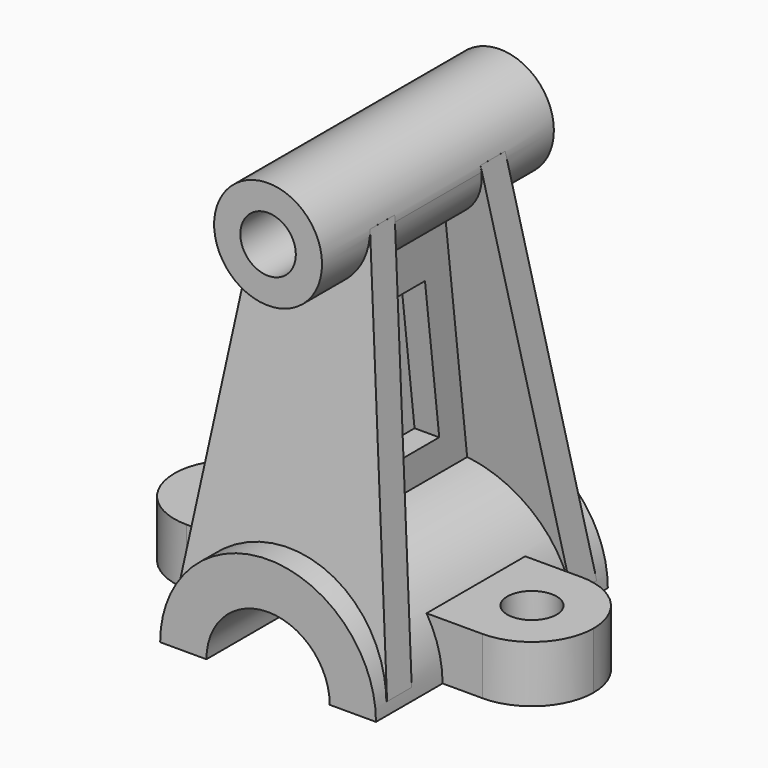
from build123d import *

# Parameters (mm, degrees)
F1_DEPTH     = 37.30625
F2_DEPTH     = 15.875
F3_R         = 15.87499
F0_R         = 13.890625
F0_R_2       = 7.14375
F4_DEPTH     = 37.30625
F6_DEPTH     = 3.175
F7_DEPTH     = 27.78125
F8_T4_DEPTH  = 515.4304915521
F8_T9_DEPTH  = 515.4304915521
F8_T14_DEPTH = 515.4304915521
F8_T19_DEPTH = 515.4304915521
F8_T24_DEPTH = 515.4304915521
F8_T29_DEPTH = 515.4304915521
F9_DEPTH     = 50.8
F10_R        = 6.35
F11_DEPTH    = 14.5721768419
F12_DEPTH    = 38.1


# Not quite as in the source:
# - a fillet or chamfer that OpenCascade refuses, or shapes differently, is made with other operations: its cross-section is extruded or revolved along the edge and cut away or added
# - a fillet or chamfer is up to 0.001 mm smaller than in the source, because OpenCascade refuses the exact size
# - a feature of the source that left no trace in its solid (it failed there, or was rolled back) is left out


with BuildPart() as f1:
    # F0 (on Front) → F1 (new body, symmetric)
    with BuildSketch(Plane.XZ):
        with BuildLine():
            Line((15.875, 0), (27.78125, 0))
            ThreePointArc((27.78125, 0), (26.7293483379, 7.5723040742), (23.6533011862, 14.5711768419))
            ThreePointArc((23.6533011862, 14.5711768419), (0, 27.78125), (-23.6533011862, 14.5711768419))
            ThreePointArc((-23.6533011862, 14.5711768419), (-26.7293483379, 7.5723040742), (-27.78125, 0))
            Line((-27.78125, 0), (-15.875, 0))
            ThreePointArc((-15.875, 0), (0, 15.875), (15.875, 0))
        make_face()
    extrude(amount=F1_DEPTH, both=True)

    # F0 (on Front) → F2 (join, symmetric)
    with BuildSketch(Plane.XZ):
        with BuildLine():
            ThreePointArc((23.6533011862, 14.5711768419), (26.7293483379, 7.5723040742), (27.78125, 0))
            Line((27.78125, 0), (53.975, 0))
            Line((53.975, 0), (53.975, 14.5711768419))
            Line((53.975, 14.5711768419), (23.6533011862, 14.5711768419))
        make_face()
        with BuildLine():
            ThreePointArc((-27.78125, 0), (-26.7293483379, 7.5723040742), (-23.6533011862, 14.5711768419))
            Line((-23.6533011862, 14.5711768419), (-53.975, 14.5711768419))
            Line((-53.975, 14.5711768419), (-53.975, 0))
            Line((-53.975, 0), (-27.78125, 0))
        make_face()
    extrude(amount=F2_DEPTH, both=True)

    # F3 (radius 15.875 in the source; OpenCascade refuses exactly that, so slightly less here)
    f3_edges = [f1.edges().sort_by_distance(p)[0] for p in [
        (53.975, -15.875, 7.285588),
        (53.975, 15.875, 7.285588),
        (-53.975, -15.875, 7.285588),
        (-53.975, 15.875, 7.285588),
    ]]
    fillet(f3_edges, radius=F3_R)



with BuildPart() as f4:
    # F0 (on Front) → F4 (new body, symmetric)
    with BuildSketch(Plane.XZ):
        with Locations((0, 99.21875)):
            Circle(F0_R)
        with Locations((0, 99.21875)):
            Circle(F0_R_2, mode=Mode.SUBTRACT)
    extrude(amount=F4_DEPTH, both=True)


with BuildPart() as f1_1:
    add(f1.part)

    add(f4.part)  # F6 merges F4
    # F5 (on Right) → F6 (join, symmetric)
    with BuildSketch(Plane.YZ):
        Polygon((-15.1982219998, 89.4941017032), (-23.1018472504, 25.1242396258), (23.1018472504, 25.1242396258), (15.1982219998, 89.4941017032), align=None)
        Polygon((-9.2232641814, 73.025), (9.2232641814, 73.025), (13.8038957065, 35.71875), (-13.8038957065, 35.71875), align=None, mode=Mode.SUBTRACT)
    extrude(amount=F6_DEPTH, both=True)

    # F5 (on Right) → F7 (join, symmetric)
    with BuildSketch(Plane.YZ):
        Polygon((-21.7467648383, 100.80625), (-33.734375, 3.175), (-25.796875, 3.175), (-23.1018472504, 25.1242396258), (-15.1982219998, 89.4941017032), (-13.8092648383, 100.80625), align=None)
        Polygon((15.1982219998, 89.4941017032), (23.1018472504, 25.1242396258), (25.796875, 3.175), (33.734375, 3.175), (21.7467648383, 100.80625), (13.8092648383, 100.80625), align=None)
    extrude(amount=F7_DEPTH, both=True)

    # F8: chamfer of 13.9762738 x 97.63125 on 2 edges, made by hand


with BuildPart() as f8_tool2:
    # F8_s3 → F8_t4 (new body)
    with BuildSketch(Plane.XZ.offset(-275.4932606144)):
        Polygon((13.8049762, 100.80625), (27.78125, 3.175), (27.78125, 100.80625), align=None)
    extrude(amount=F8_T4_DEPTH)

    split(bisect_by=Plane.XY.offset(14.5711768419), keep=Keep.TOP)


with BuildPart() as f1_2:
    add(f1_1.part)

    # F8_t1: cut F8_tool2
    add(f8_tool2.part, mode=Mode.SUBTRACT)


with BuildPart() as f8_tool7:
    # F8_s8 → F8_t9 (new body)
    with BuildSketch(Plane.XZ.offset(-275.4932606144)):
        Polygon((13.8049762, 100.80625), (27.78125, 3.175), (27.78125, 100.80625), align=None)
    extrude(amount=F8_T9_DEPTH)

    split(bisect_by=Plane.XZ.offset(-15.875), keep=Keep.BOTTOM)


with BuildPart() as f1_3:
    add(f1_2.part)

    # F8_t6: cut F8_tool7
    add(f8_tool7.part, mode=Mode.SUBTRACT)


with BuildPart() as f8_tool12:
    # F8_s13 → F8_t14 (new body)
    with BuildSketch(Plane.XZ.offset(-275.4932606144)):
        Polygon((13.8049762, 100.80625), (27.78125, 3.175), (27.78125, 100.80625), align=None)
    extrude(amount=F8_T14_DEPTH)

    split(bisect_by=Plane.XZ.offset(15.875), keep=Keep.TOP)


with BuildPart() as f1_4:
    add(f1_3.part)

    # F8_t11: cut F8_tool12
    add(f8_tool12.part, mode=Mode.SUBTRACT)


with BuildPart() as f8_tool17:
    # F8_s18 → F8_t19 (new body)
    with BuildSketch(Plane.XZ.offset(-239.9372309377)):
        Polygon((-13.8049762, 100.80625), (-27.78125, 3.175), (-27.78125, 100.80625), align=None)
    extrude(amount=F8_T19_DEPTH)

    split(bisect_by=Plane.XY.offset(14.5711768419), keep=Keep.TOP)


with BuildPart() as f1_5:
    add(f1_4.part)

    # F8_t16: cut F8_tool17
    add(f8_tool17.part, mode=Mode.SUBTRACT)


with BuildPart() as f8_tool22:
    # F8_s23 → F8_t24 (new body)
    with BuildSketch(Plane.XZ.offset(-239.9372309377)):
        Polygon((-13.8049762, 100.80625), (-27.78125, 3.175), (-27.78125, 100.80625), align=None)
    extrude(amount=F8_T24_DEPTH)

    split(bisect_by=Plane.XZ.offset(-15.875), keep=Keep.BOTTOM)


with BuildPart() as f1_6:
    add(f1_5.part)

    # F8_t21: cut F8_tool22
    add(f8_tool22.part, mode=Mode.SUBTRACT)


with BuildPart() as f8_tool27:
    # F8_s28 → F8_t29 (new body)
    with BuildSketch(Plane.XZ.offset(-239.9372309377)):
        Polygon((-13.8049762, 100.80625), (-27.78125, 3.175), (-27.78125, 100.80625), align=None)
    extrude(amount=F8_T29_DEPTH)

    split(bisect_by=Plane.XZ.offset(15.875), keep=Keep.TOP)


with BuildPart() as f1_7:
    add(f1_6.part)

    # F8_t26: cut F8_tool27
    add(f8_tool27.part, mode=Mode.SUBTRACT)

    # F0 (on Front) → F9 (cut, symmetric)
    with BuildSketch(Plane.XZ):
        with BuildLine():
            Line((-15.875, 0), (15.875, 0))
            ThreePointArc((15.875, 0), (0, 15.875), (-15.875, 0))
        make_face()
    extrude(amount=F9_DEPTH, both=True, mode=Mode.SUBTRACT)

    # F10 (on face) → F11 (cut, through all)
    with BuildSketch(Plane.XY.offset(14.5711768419)):
        with Locations((-38.1, 0)):
            Circle(F10_R)
        with Locations((38.1, 0)):
            Circle(F10_R)
    extrude(amount=-F11_DEPTH, mode=Mode.SUBTRACT)

    # F0 (on Front) → F12 (cut, symmetric)
    with BuildSketch(Plane.XZ):
        with Locations((0, 99.21875)):
            Circle(F0_R_2)
    extrude(amount=F12_DEPTH, both=True, mode=Mode.SUBTRACT)


solid = f1_7.part
